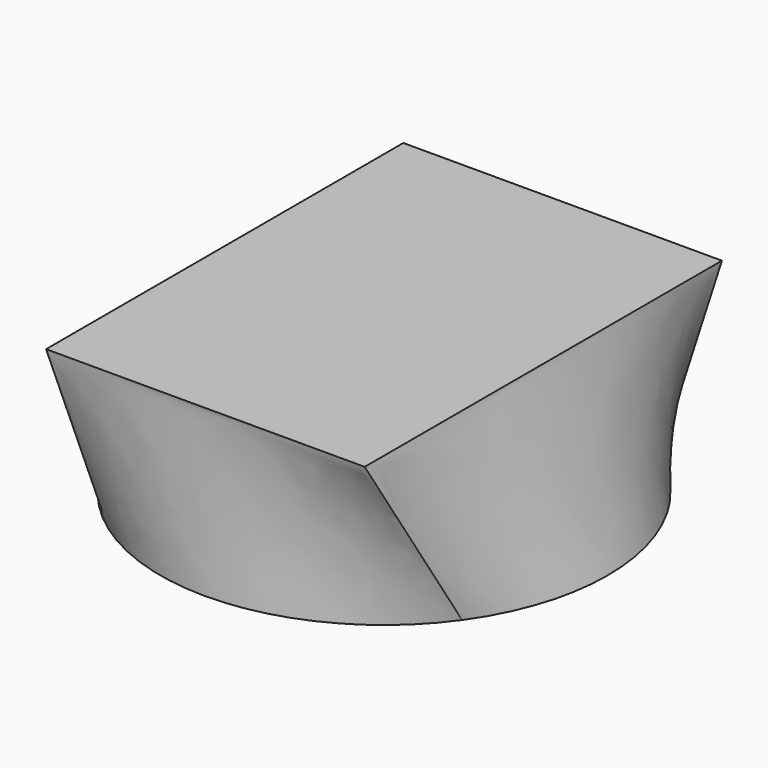
from build123d import *

# Parameters (mm, degrees)
F2_W = 48.1534339488
F2_H = 67.4888566136


# Not quite as in the source:
# - the arcs of a loft's sections are written as splines that run evenly, so that the points pair up as in the source's solid


with BuildPart() as f3:
    # F0 (on Top) → F3 section 0
    with BuildSketch(Plane.XY):
        with BuildLine():
            add(Edge.make_bspline(
                [(-19.6366312529, -27.5214804497), (-17.8353545697, -28.8066949598), (-15.9075429758, -29.9144718089), (-11.8727458368, -31.7326874599), (-9.7658600599, -32.4430813028), (-5.4538741397, -33.4392105768), (-3.2488806187, -33.7249213766), (1.174586882, -33.8606835842), (3.3929514827, -33.710731635), (7.7579091885, -32.9809095107), (9.9043943614, -32.4010573819), (14.0430993957, -30.8336975806), (16.0352169193, -29.8462286643), (19.7886211685, -27.5015639443), (21.5498150836, -26.1444261171), (24.7736773273, -23.1125606286), (26.2362659395, -21.4379079362), (27.5214804497, -19.6366312529)],
                knots=[0, 0, 0, 0, 0.125, 0.125, 0.25, 0.25, 0.375, 0.375, 0.5, 0.5, 0.625, 0.625, 0.75, 0.75, 0.875, 0.875, 1, 1, 1, 1], degree=3))
            add(Edge.make_bspline(
                [(27.5214804497, -19.6366312529), (28.8066949598, -17.8353545697), (29.9144718089, -15.9075429758), (31.7326874599, -11.8727458368), (32.4430813028, -9.7658600599), (33.4392105768, -5.4538741397), (33.7249213766, -3.2488806187), (33.8606835842, 1.174586882), (33.710731635, 3.3929514827), (32.9809095107, 7.7579091885), (32.4010573819, 9.9043943614), (30.8336975806, 14.0430993957), (29.8462286643, 16.0352169193), (27.5015639443, 19.7886211685), (26.1444261171, 21.5498150836), (23.1125606286, 24.7736773273), (21.4379079362, 26.2362659395), (19.6366312529, 27.5214804497)],
                knots=[0, 0, 0, 0, 0.125, 0.125, 0.25, 0.25, 0.375, 0.375, 0.5, 0.5, 0.625, 0.625, 0.75, 0.75, 0.875, 0.875, 1, 1, 1, 1], degree=3))
            add(Edge.make_bspline(
                [(19.6366312529, 27.5214804497), (17.8353545697, 28.8066949598), (15.9075429758, 29.9144718089), (11.8727458368, 31.7326874599), (9.7658600599, 32.4430813028), (5.4538741397, 33.4392105768), (3.2488806187, 33.7249213766), (-1.174586882, 33.8606835842), (-3.3929514827, 33.710731635), (-7.7579091885, 32.9809095107), (-9.9043943614, 32.4010573819), (-14.0430993957, 30.8336975806), (-16.0352169193, 29.8462286643), (-19.7886211685, 27.5015639443), (-21.5498150836, 26.1444261171), (-24.7736773273, 23.1125606286), (-26.2362659395, 21.4379079362), (-27.5214804497, 19.6366312529)],
                knots=[0, 0, 0, 0, 0.125, 0.125, 0.25, 0.25, 0.375, 0.375, 0.5, 0.5, 0.625, 0.625, 0.75, 0.75, 0.875, 0.875, 1, 1, 1, 1], degree=3))
            add(Edge.make_bspline(
                [(-27.5214804497, 19.6366312529), (-28.8066949598, 17.8353545697), (-29.9144718089, 15.9075429758), (-31.7326874599, 11.8727458368), (-32.4430813028, 9.7658600599), (-33.4392105768, 5.4538741397), (-33.7249213766, 3.2488806187), (-33.8606835842, -1.174586882), (-33.710731635, -3.3929514827), (-32.9809095107, -7.7579091885), (-32.4010573819, -9.9043943614), (-30.8336975806, -14.0430993957), (-29.8462286643, -16.0352169193), (-27.5015639443, -19.7886211685), (-26.1444261171, -21.5498150836), (-23.1125606286, -24.7736773273), (-21.4379079362, -26.2362659395), (-19.6366312529, -27.5214804497)],
                knots=[0, 0, 0, 0, 0.125, 0.125, 0.25, 0.25, 0.375, 0.375, 0.5, 0.5, 0.625, 0.625, 0.75, 0.75, 0.875, 0.875, 1, 1, 1, 1], degree=3))
        make_face()
    # F2 (on offset) → F3 section 1
    with BuildSketch(Plane.XY.offset(25)):
        Rectangle(F2_W, F2_H)
    loft(ruled=True)


solid = f3.part
